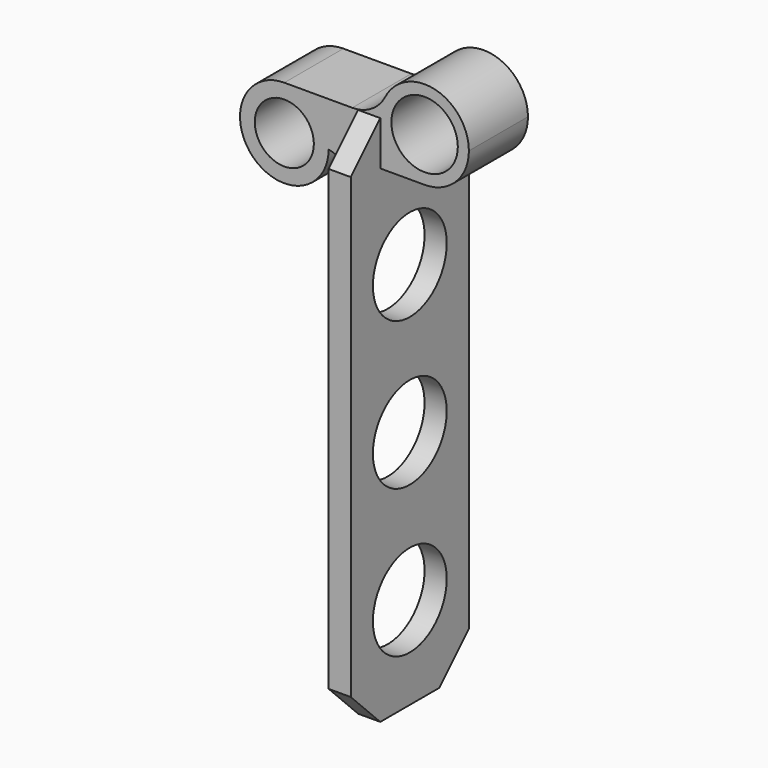
from build123d import *

# Parameters (mm, degrees)
F0_R          = 8
F0_R_2        = 9
F1_DEPTH      = 20
F2_W          = 6
F2_H          = 144
F3_DEPTH      = 10
F3_DEPTH_BACK = 30
F4_SIZE       = 10
F5_T1_DEPTH   = 20
F6_R          = 12.5
F7_DEPTH      = 6


# Not quite as in the source:
# - a fillet or chamfer that OpenCascade refuses, or shapes differently, is made with other operations: its cross-section is extruded or revolved along the edge and cut away or added


with BuildPart() as f1:
    # F0 (on Front) → F1 (new body)
    with BuildSketch(Plane.XZ):
        with BuildLine():
            ThreePointArc((0, 12), (-8.4852813742, -8.4852813742), (12, 0))
            ThreePointArc((12, 0), (8.4852813742, 8.4852813742), (0, 12))
        make_face()
        Circle(F0_R, mode=Mode.SUBTRACT)
        with BuildLine():
            ThreePointArc((0, 12), (8.4852813742, 8.4852813742), (12, 0))
            Line((12, 0), (38, 0))
            ThreePointArc((38, 0), (29.5147186258, 3.5147186258), (26, 12))
            Line((26, 12), (0, 12))
        make_face()
        with BuildLine():
            ThreePointArc((26, 12), (29.5147186258, 3.5147186258), (38, 0))
            ThreePointArc((38, 0), (46.4852813742, 3.5147186258), (50, 12))
            ThreePointArc((50, 12), (38, 24), (26, 12))
        make_face()
        with Locations((38, 12)):
            Circle(F0_R_2, mode=Mode.SUBTRACT)
    extrude(amount=F1_DEPTH)

    # F2 (on face) → F3 (join, two sides)
    with BuildSketch(Plane.XZ.offset(20)) as f3_sk:
        with Locations((23, -60)):
            Rectangle(F2_W, F2_H)
    extrude(amount=F3_DEPTH)
    extrude(f3_sk.sketch, amount=-F3_DEPTH_BACK)

    # F4
    f4_edges = [f1.edges().sort_by_distance(p)[0] for p in [
        (23, -30, 12),
        (23, 10, 12),
        (23, -30, -132),
        (23, 10, -132),
    ]]
    chamfer(f4_edges, length=F4_SIZE)

    # F5: fillet of radius 10 on 2 edges, made by hand

    # F5_s2 → F5_t1 (join)
    with BuildSketch(Plane.XZ):
        with BuildLine():
            ThreePointArc((18.4040820577, 12), (23.6264117364, 13.4719713458), (27.311317486, 17.4545454545))
            ThreePointArc((27.311317486, 17.4545454545), (26.3324340549, 14.8049785946), (26, 12))
            Line((26, 12), (18.4040820577, 12))
        make_face()
        with BuildLine():
            ThreePointArc((20, -9.7979589711), (17.7459666924, -3.4734036508), (12, 0))
            Line((12, 0), (20, 0))
            Line((20, 0), (20, -9.7979589711))
        make_face()
    extrude(amount=F5_T1_DEPTH)

    # F6 (on face) → F7 (cut, through all)
    with BuildSketch(Plane(origin=(20, 0, 0), x_dir=(0, -1, 0), z_dir=(-1, 0, 0))):
        with Locations((10, -107)):
            Circle(F6_R)
        with Locations((10, -67)):
            Circle(F6_R)
        with Locations((10, -27)):
            Circle(F6_R)
    extrude(amount=-F7_DEPTH, mode=Mode.SUBTRACT)


solid = f1.part
